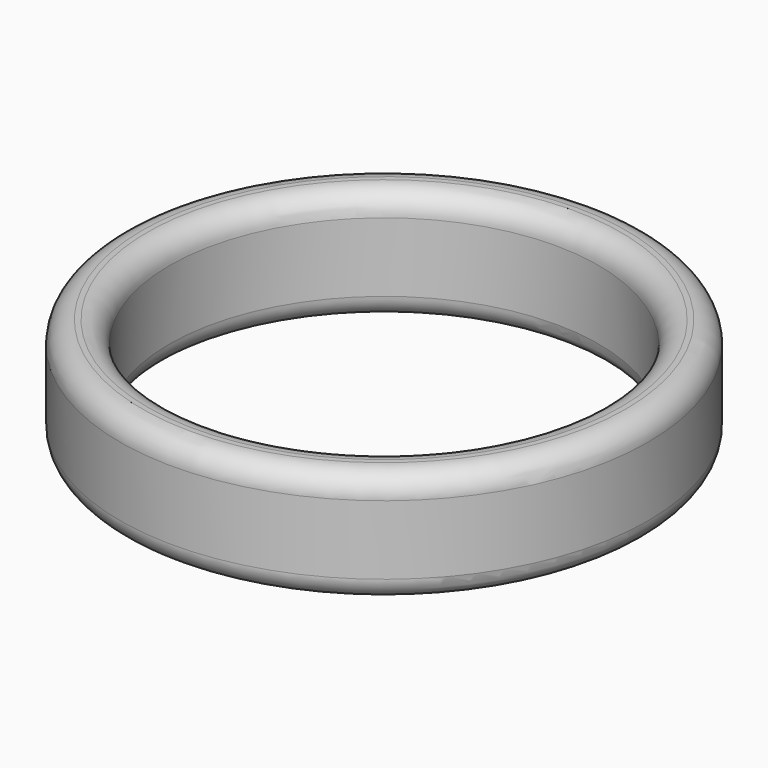
from build123d import *

# Parameters (mm, degrees)
F0_R     = 59.8414566133
F0_R_2   = 48.6676693488
F3_DEPTH = 25
F7_T     = -2.5


# Not quite as in the source:
# - a fillet or chamfer that OpenCascade refuses, or shapes differently, is made with other operations: its cross-section is extruded or revolved along the edge and cut away or added
# - the program builds the solid bodies; features that only make, move or delete a surface that nothing else refers to are left out


with BuildPart() as f3:
    # F0 (on Top) → F3 (new body)
    with BuildSketch(Plane.XY):
        Circle(F0_R)
        Circle(F0_R_2, mode=Mode.SUBTRACT)
    extrude(amount=F3_DEPTH)

    # F7
    f7_openings = [f3.faces().sort_by_distance(p)[0] for p in [
        (-58.148885, 0, 0),
    ]]
    offset(amount=F7_T, openings=f7_openings)

    # F8: fillet of radius 5 on 3 edges, made by hand

    # F8_s1 → F8_t2 (revolve, cut)
    with BuildSketch(Plane.XZ):
        with BuildLine():
            ThreePointArc((59.8414566133, 4.3301270189), (59.1715836322, 1.8301270189), (57.3414566133, 0))
            Line((57.3414566133, 0), (59.8414566133, 0))
            Line((59.8414566133, 0), (59.8414566133, 4.3301270189))
        make_face()
    revolve(axis=Axis((0, 0, 0), (0, 0, 1)), mode=Mode.SUBTRACT)

    # F8_s3 → F8_t4 (revolve, cut)
    with BuildSketch(Plane.XZ):
        with BuildLine():
            ThreePointArc((59.8414566133, 20), (58.3769905192, 23.5355339059), (54.8414566133, 25))
            Line((54.8414566133, 25), (59.8414566133, 25))
            Line((59.8414566133, 25), (59.8414566133, 20))
        make_face()
    revolve(axis=Axis((0, 0, 25), (0, 0, 1)), mode=Mode.SUBTRACT)

    # F9: fillet of radius 5 on 3 edges, made by hand

    # F9_s1 → F9_t2 (revolve, cut)
    with BuildSketch(Plane.XZ):
        with BuildLine():
            ThreePointArc((48.6676693488, 4.3301270189), (49.3375423299, 1.8301270189), (51.1676693488, 0))
            Line((51.1676693488, 0), (48.6676693488, 0))
            Line((48.6676693488, 0), (48.6676693488, 4.3301270189))
        make_face()
    revolve(axis=Axis((0, 0, 0), (0, 0, 1)), mode=Mode.SUBTRACT)

    # F9_s3 → F9_t4 (revolve, cut)
    with BuildSketch(Plane.XZ):
        with BuildLine():
            ThreePointArc((53.6676693488, 25), (50.1321354429, 23.5355339059), (48.6676693488, 20))
            Line((48.6676693488, 20), (48.6676693488, 25))
            Line((48.6676693488, 25), (53.6676693488, 25))
        make_face()
    revolve(axis=Axis((0, 0, 25), (0, 0, 1)), mode=Mode.SUBTRACT)


solid = f3.part
